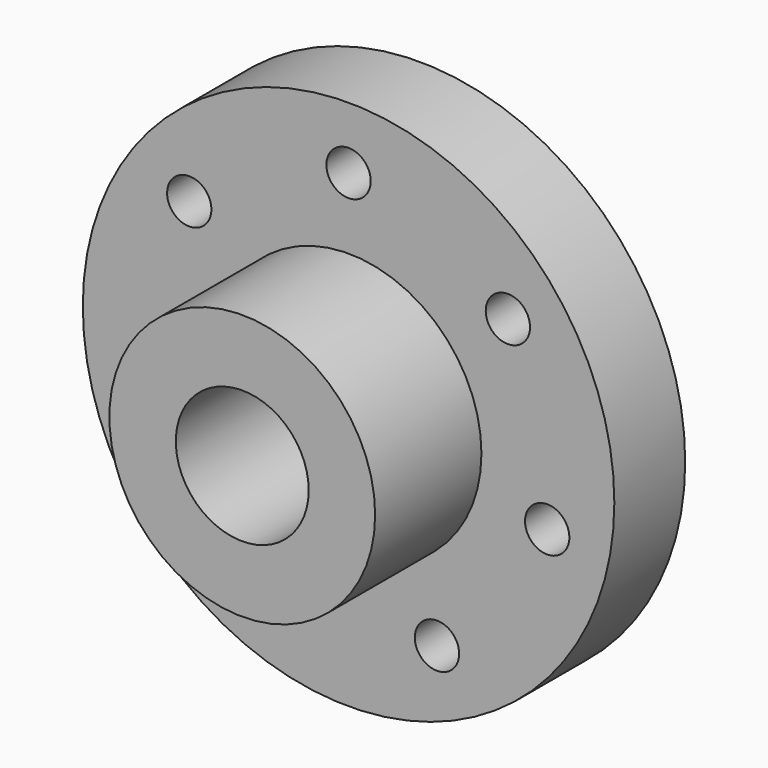
from build123d import *

# Parameters (mm, degrees)
F0_R            = 38.1
F0_R_2          = 19.05
F1_DEPTH        = 12.7
F0_R_3          = 9.525
F2_DEPTH        = 31.75
F3_R            = 3.175
F4_DEPTH        = 12.701
F4_COPIES_COUNT = 7


# Not quite as in the source:
# - a pattern or mirror of a feature is missing from the dataset's text; its kind, count and spacing are read off the source's solid


with BuildPart() as f1:
    # F0 (on Front) → F1 (new body)
    with BuildSketch(Plane.XZ):
        Circle(F0_R)
        Circle(F0_R_2, mode=Mode.SUBTRACT)
    extrude(amount=F1_DEPTH)

    # F0 (on Front) → F2 (join)
    with BuildSketch(Plane.XZ):
        Circle(F0_R_2)
        Circle(F0_R_3, mode=Mode.SUBTRACT)
    extrude(amount=F2_DEPTH)

    # F3 (on face) → F4 (cut, through all)
    with BuildSketch(Plane.XZ.offset(12.7)):
        with Locations((0, 29.21)):
            Circle(F3_R)
    f4 = extrude(amount=-F4_DEPTH, mode=Mode.SUBTRACT)

    # F4_copies: F4 ×7 about axis
    f4_copies_axis = Axis((0, 0, 0), (0, 1, 0))
    for i in range(1, F4_COPIES_COUNT):
        add(f4.rotate(f4_copies_axis, i * 360 / F4_COPIES_COUNT), mode=Mode.SUBTRACT)


solid = f1.part
